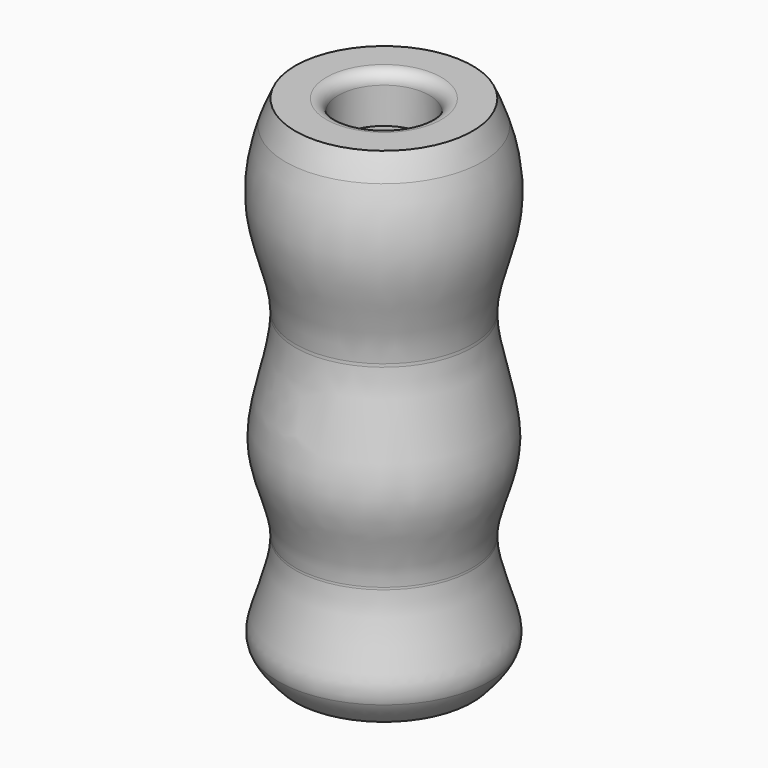
from build123d import *

# Parameters (mm, degrees)
F0_W = 5.975
F0_H = 10
F2_R = 4.99999
F3_R = 5


# Not quite as in the source:
# - a fillet or chamfer is up to 0.001 mm smaller than in the source, because OpenCascade refuses the exact size


with BuildPart() as f1:
    # F0 (on Front) → F1 (revolve)
    with BuildSketch(Plane.XZ):
        with BuildLine():
            Line((-31.025, 73.7897304978), (-26.025, 73.7897304978))
            Line((-26.025, 73.7897304978), (-26.025, 98.7897304978))
            Line((-26.025, 98.7897304978), (-19, 98.7897304978))
            Line((-19, 98.7897304978), (-19, 118.7897304978))
            Line((-19, 118.7897304978), (-37, 118.7897304978))
            Line((-37, 118.7897304978), (-37, 108.7897304978))
            Line((-37, 108.7897304978), (-41.0849433686, 108.7897304978))
            add(Edge.make_bspline(
                [(-41.0849433686, 108.7897304978), (-45.1725468115, 96.8054937838), (-47.4207058778, 72.2712183097), (-37.1834587857, 52.689037564), (-37, 40.4585758234)],
                knots=[0.0406718055, 0.0406718055, 0.0406718055, 0.0406718055, 0.1878766182, 0.3513528172, 0.3513528172, 0.3513528172, 0.3513528172], degree=3))
            add(Edge.make_bspline(
                [(-37, 40.4585758234), (-36.9936533209, 40.0354681691), (-36.9935338048, 39.6100548134), (-37, 39.182199225)],
                knots=[0.3513528172, 0.3513528172, 0.3513528172, 0.3513528172, 0.3570082072, 0.3570082072, 0.3570082072, 0.3570082072], degree=3))
            Line((-37, 39.182199225), (-37, -41.7443042648))
            add(Edge.make_bspline(
                [(-37, -41.7443042648), (-36.9955207148, -42.05056935), (-36.9955908911, -42.357808797), (-37, -42.6659036208)],
                knots=[0.7164749618, 0.7164749618, 0.7164749618, 0.7164749618, 0.7208378699, 0.7208378699, 0.7208378699, 0.7208378699], degree=3))
            Line((-37, -42.6659036208), (-37, -81.2102695022))
            Line((-37, -81.2102695022), (-31.025, -81.2102695022))
            Line((-31.025, -81.2102695022), (-31.025, -74.6120512486))
            Line((-31.025, -74.6120512486), (-31.025, 73.7897304978))
        make_face()
        with Locations((-34.0125, -86.2102695022)):
            Rectangle(F0_W, F0_H)
        with BuildLine():
            Line((-37, 108.7897304978), (-37, 118.7897304978))
            add(Edge.make_bspline(
                [(-37, 118.7897304978), (-38.5954580496, 115.4395246778), (-39.9555630892, 112.1009031194), (-41.0849433686, 108.7897304978)],
                knots=[0, 0, 0, 0, 0.0406718055, 0.0406718055, 0.0406718055, 0.0406718055], degree=3))
            Line((-41.0849433686, 108.7897304978), (-37, 108.7897304978))
        make_face()
        with BuildLine():
            Line((-44.2141639133, -81.2102695022), (-37, -81.2102695022))
            Line((-37, -81.2102695022), (-37, -42.6659036208))
            add(Edge.make_bspline(
                [(-37, -42.6659036208), (-37.1579517608, -53.7030816804), (-45.0079078812, -70.3382328063), (-45.133027455, -78.7563351769), (-44.2141639133, -81.2102695022)],
                knots=[0.7208378699, 0.7208378699, 0.7208378699, 0.7208378699, 0.8771345363, 0.9350969036, 0.9350969036, 0.9350969036, 0.9350969036], degree=3))
        make_face()
        with BuildLine():
            Line((-37, -91.2102695022), (-37, -81.2102695022))
            Line((-37, -81.2102695022), (-44.2141639133, -81.2102695022))
            add(Edge.make_bspline(
                [(-44.2141639133, -81.2102695022), (-43.1852706536, -83.9580512704), (-40.9618393029, -86.9272963181), (-37, -91.2102695022)],
                knots=[0.9350969036, 0.9350969036, 0.9350969036, 0.9350969036, 1, 1, 1, 1], degree=3))
        make_face()
        with BuildLine():
            Line((-37, -41.7443042648), (-37, -42.6659036208))
            add(Edge.make_bspline(
                [(-37, -41.7443042648), (-36.9955207148, -42.05056935), (-36.9955908911, -42.357808797), (-37, -42.6659036208)],
                knots=[0.7164749618, 0.7164749618, 0.7164749618, 0.7164749618, 0.7208378699, 0.7208378699, 0.7208378699, 0.7208378699], degree=3))
        make_face()
        with BuildLine():
            add(Edge.make_bspline(
                [(-37, 40.4585758234), (-36.9936533209, 40.0354681691), (-36.9935338048, 39.6100548134), (-37, 39.182199225)],
                knots=[0.3513528172, 0.3513528172, 0.3513528172, 0.3513528172, 0.3570082072, 0.3570082072, 0.3570082072, 0.3570082072], degree=3))
            Line((-37, 40.4585758234), (-37, 39.182199225))
        make_face()
        with BuildLine():
            add(Edge.make_bspline(
                [(-37, 39.182199225), (-37.2201394503, 24.6159989291), (-51.882227124, -7.864116597), (-37.1713836413, -30.0261788456), (-37, -41.7443042648)],
                knots=[0.3570082072, 0.3570082072, 0.3570082072, 0.3570082072, 0.5495440671, 0.7164749618, 0.7164749618, 0.7164749618, 0.7164749618], degree=3))
            Line((-37, -41.7443042648), (-37, 39.182199225))
        make_face()
    revolve(axis=Axis((0, 0, -7.4881389737), (0, 0, -1)))

    # F2 (radius 5 in the source; OpenCascade refuses exactly that, so slightly less here)
    f2_edges = [f1.edges().sort_by_distance(p)[0] for p in [
        (26.025, 0, 73.78973),
    ]]
    fillet(f2_edges, radius=F2_R)

    # F3
    f3_edges = [f1.edges().sort_by_distance(p)[0] for p in [
        (19, 0, 118.78973),
        (31.025, 0, -91.21027),
    ]]
    fillet(f3_edges, radius=F3_R)


with BuildPart() as f4_1:
    # F4: copy of F1
    add(f1.part)


solid = Compound([f1.part, f4_1.part])
